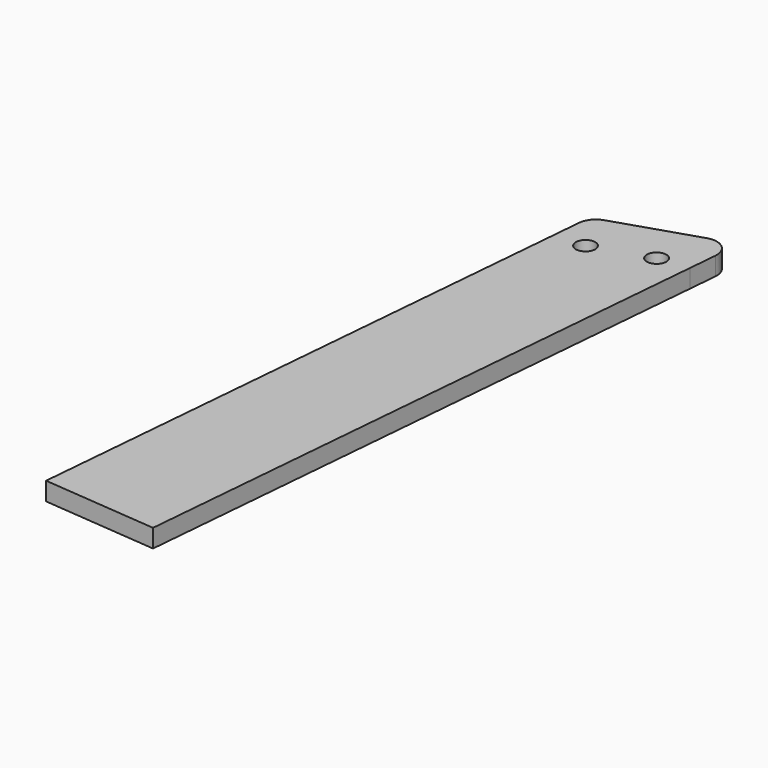
from build123d import *

# Parameters (mm, degrees)
F0_R     = 1.6
F1_DEPTH = 3


with BuildPart() as f1:
    # F0 (on Top) → F1 (new body)
    with BuildSketch(Plane.XY):
        with BuildLine():
            Line((-19.4697175733, -4.5393385149), (-19.4718945337, -4.5642212863))
            Line((-19.4718945337, -4.5642212863), (-28.1188425534, -103.3992894107))
            Line((-28.1188425534, -103.3992894107), (-9.1911432897, -105.0552485229))
            Line((-9.1911432897, -105.0552485229), (-0.4755690149, -5.4357787137))
            Line((-0.4755690149, -5.4357787137), (-0.0637739547, -0.7289396381))
            ThreePointArc((-0.0637739547, -0.7289396381), (-1.1824461608, 1.8784665345), (-3.9736495146, 2.3875620971))
            Line((-3.9736495146, 2.3875620971), (-17.4024249446, -1.9457712363))
            ThreePointArc((-17.4024249446, -1.9457712363), (-18.8270724233, -2.930893855), (-19.4697175733, -4.5393385149))
        make_face()
        with Locations((-14.8408756973, -9)):
            Circle(F0_R, mode=Mode.SUBTRACT)
        with Locations((-5.5440311689, -6)):
            Circle(F0_R, mode=Mode.SUBTRACT)
    extrude(amount=F1_DEPTH)


solid = f1.part
